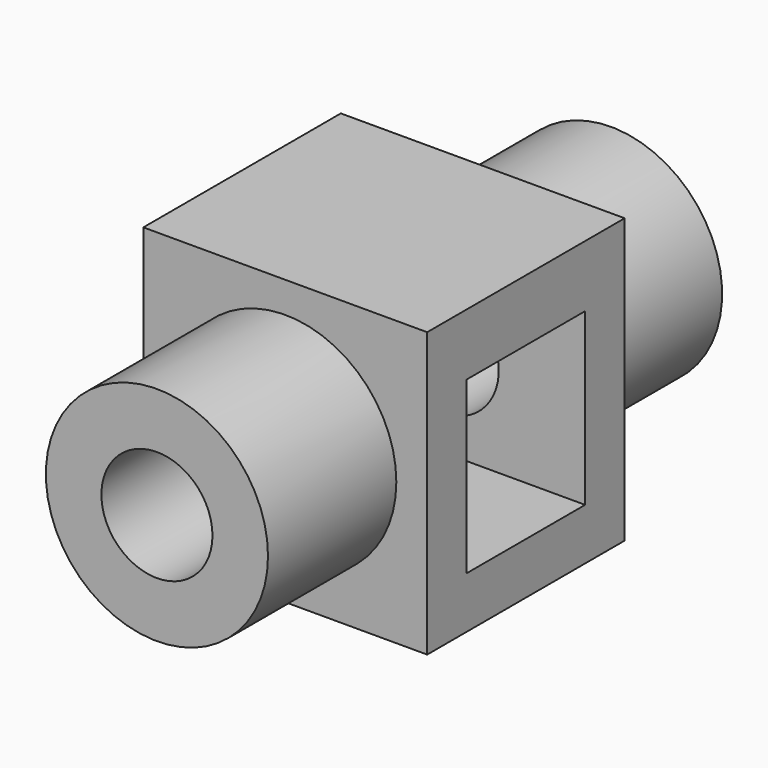
from build123d import *
from build123d import SkipClean  # not in build123d's __all__

# Parameters (mm, degrees)
F0_W      = 46
F0_H      = 40
F1_DEPTH  = 46
F2_W      = 24
F2_H      = 27.6410613805
F3_DEPTH  = 46
F4_R      = 9
F6_DEPTH  = 46
F5_R      = 18
F7_DEPTH  = 26
F8_R      = 9
F9_DEPTH  = 26
F10_R     = 18
F10_R_2   = 9
F11_DEPTH = 26


with BuildPart() as f1:
    # F0 (on Top) → F1 (new body)
    with BuildSketch(Plane.XY):
        with Locations((23, -20)):
            Rectangle(F0_W, F0_H)
    extrude(amount=F1_DEPTH)

    # F2 (on face) → F3 (cut)
    with BuildSketch(Plane.YZ.offset(46)):
        with Locations((-20, 22.1794693097)):
            Rectangle(F2_W, F2_H)
    extrude(amount=-F3_DEPTH, mode=Mode.SUBTRACT)

    # F4 (on face) → F6 (cut)
    with BuildSketch(Plane(origin=(0, 0, 0), x_dir=(-1, 0, 0), z_dir=(0, 1, 0))):
        with Locations((-23, 23)):
            Circle(F4_R)
    extrude(amount=-F6_DEPTH, mode=Mode.SUBTRACT)

    # F5 (on face) → F7 (join)
    with BuildSketch(Plane(origin=(0, 0, 0), x_dir=(-1, 0, 0), z_dir=(0, 1, 0))):
        with Locations((-23, 23)):
            Circle(F5_R)
    extrude(amount=F7_DEPTH)

    # F8 (on face) → F9 (cut)
    with BuildSketch(Plane(origin=(0, 26, 0), x_dir=(-1, 0, 0), z_dir=(0, 1, 0))):
        with Locations((-23, 23)):
            Circle(F8_R)
    extrude(amount=-F9_DEPTH, mode=Mode.SUBTRACT)

    # F10 (on face) → F11 (join)
    with BuildSketch(Plane.XZ.offset(40)):
        with Locations((23, 23)):
            Circle(F10_R)
        with Locations((23, 23)):
            Circle(F10_R_2, mode=Mode.SUBTRACT)
    with SkipClean():  # cleaning this boolean's faces spoils the solid; the shape is the same uncleaned
        extrude(amount=F11_DEPTH)


solid = f1.part
